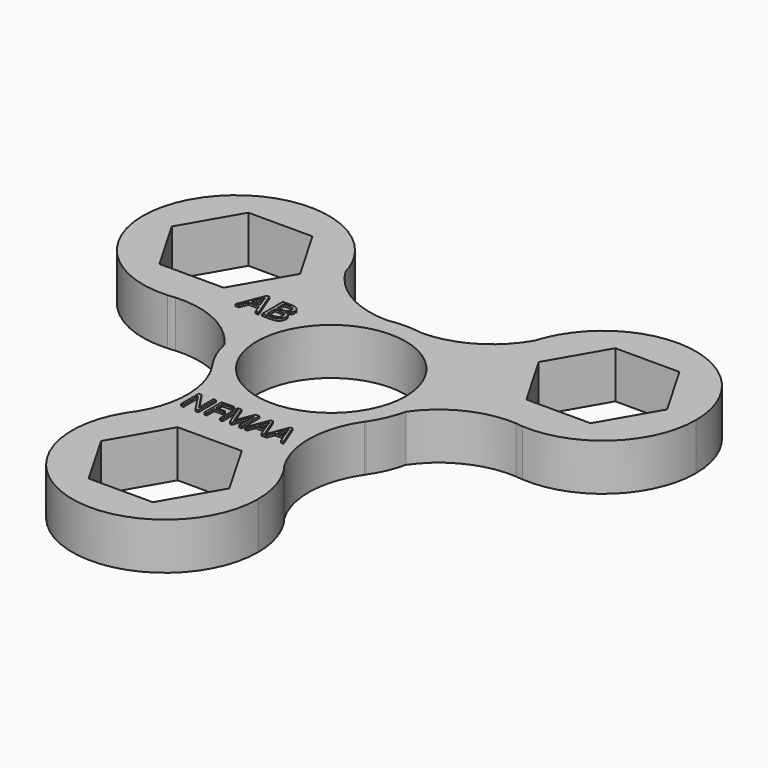
from build123d import *

# Parameters (mm, degrees)
F1_TEXT_SIZE = 4.5833333085
F2_DEPTH     = 7.3
F0_R         = 11.1353903362
F3_DEPTH     = 7
F4_TEXT_SIZE = 5.4166671665
F5_DEPTH     = 7.3


# Not quite as in the source:
# - Text() gives the source's letters only with a copy of the font that has no kerning and outlines rounded to 1/6400 em; it was checked with that copy


with BuildPart() as f2:
    # F1 (on Top) → F2 (new body)
    with BuildSketch(Plane.XY):
        with Locations((-8.2499992568, -18.2999996468)):
            Text('NFMAA', F1_TEXT_SIZE, font='Open Sans', text_align=(TextAlign.LEFT, TextAlign.BOTTOM))
    extrude(amount=F2_DEPTH)


with BuildPart() as f3:
    # F0 (on Top) → F3 (new body)
    with BuildSketch(Plane.XY):
        with BuildLine():
            ThreePointArc((13.5864677481, -3.0033933621), (13.8322264387, -1.5106254678), (13.9144700782, 0))
            ThreePointArc((13.9144700782, 0), (10.6851705077, 8.9128900351), (2.4961971103, 13.6887354253))
            ThreePointArc((2.4961971103, 13.6887354253), (1.2428155139, 13.7431823355), (0, 13.9144700782))
            ThreePointArc((0, 13.9144700782), (-1.2734696294, 13.7344813122), (-2.558322411, 13.6772608368))
            ThreePointArc((-2.558322411, 13.6772608368), (-11.6070934538, 7.6738425258), (-13.5864677481, -3.0033933621))
            ThreePointArc((-13.5864677481, -3.0033933621), (-12.2930583167, -5.3260981533), (-11.4830526526, -7.8582427638))
            ThreePointArc((-11.4830526526, -7.8582427638), (-11.4395938725, -7.9206308518), (-11.3964893616, -7.9832642313))
            ThreePointArc((-11.3964893616, -7.9832642313), (0, -13.9144700782), (11.3964893616, -7.9832642313))
            ThreePointArc((11.3964893616, -7.9832642313), (11.4395938725, -7.9206308518), (11.4830526526, -7.8582427638))
            ThreePointArc((11.4830526526, -7.8582427638), (12.2930583167, -5.3260981533), (13.5864677481, -3.0033933621))
        make_face()
        Circle(F0_R, mode=Mode.SUBTRACT)
        with BuildLine():
            ThreePointArc((2.4961971103, 13.6887354253), (10.6851705077, 8.9128900351), (13.9144700782, 0))
            ThreePointArc((13.9144700782, 0), (13.8322264387, -1.5106254678), (13.5864677481, -3.0033933621))
            ThreePointArc((13.5864677481, -3.0033933621), (18.7682974416, 1.4209787448), (25.4552118556, 2.7292612574))
            ThreePointArc((25.4552118556, 2.7292612574), (15.7241567662, 9.0088698377), (14.1162936282, 20.4780325449))
            ThreePointArc((14.1162936282, 20.4780325449), (9.2191414593, 15.5209334854), (2.4961971103, 13.6887354253))
        make_face()
        with BuildLine():
            ThreePointArc((0, 13.9144700782), (1.2428155139, 13.7431823355), (2.4961971103, 13.6887354253))
            ThreePointArc((2.4961971103, 13.6887354253), (1.2531915403, 13.8579215079), (0, 13.9144700782))
        make_face()
        with BuildLine():
            ThreePointArc((11.4830526526, -7.8582427638), (12.7676389343, -5.5317152493), (13.5864677481, -3.0033933621))
            ThreePointArc((13.5864677481, -3.0033933621), (12.2930583167, -5.3260981533), (11.4830526526, -7.8582427638))
        make_face()
        with BuildLine():
            ThreePointArc((-2.558322411, 13.6772608368), (-1.2734696294, 13.7344813122), (0, 13.9144700782))
            ThreePointArc((0, 13.9144700782), (-1.2846479851, 13.8550408556), (-2.558322411, 13.6772608368))
        make_face()
        with BuildLine():
            ThreePointArc((15.3229415527, 23.3225313582), (14.8017809107, 21.8654279382), (14.1162936282, 20.4780325449))
            ThreePointArc((14.1162936282, 20.4780325449), (15.7241567662, 9.0088698377), (25.4552118556, 2.7292612574))
            ThreePointArc((25.4552118556, 2.7292612574), (26.0018090129, 2.6832452791), (26.5460682638, 2.6149240491))
            ThreePointArc((26.5460682638, 2.6149240491), (36.9640624183, 6.3464255382), (41.3644709454, 16.5000017732))
            ThreePointArc((41.3644709454, 16.5000017732), (30.9763923364, 29.9602038803), (15.3229415527, 23.3225313582))
        make_face()
        Polygon((17.8500022739, 16.5000017732), (22.6500015706, 24.8138444314), (32.2500001639, 24.8138444314), (37.0499994606, 16.5000017732), (32.2500001639, 8.1861591151), (22.6500015706, 8.1861591151), align=None, mode=Mode.SUBTRACT)
        with BuildLine():
            ThreePointArc((15.3229415527, 23.3225313582), (14.6404164966, 21.9338793766), (14.1162936282, 20.4780325449))
            ThreePointArc((14.1162936282, 20.4780325449), (14.8017809107, 21.8654279382), (15.3229415527, 23.3225313582))
        make_face()
        with BuildLine():
            ThreePointArc((11.3964893616, -7.9832642313), (11.4399417956, -7.9208717494), (11.4830526526, -7.8582427638))
            ThreePointArc((11.4830526526, -7.8582427638), (11.4395938725, -7.9206308518), (11.3964893616, -7.9832642313))
        make_face()
        with BuildLine():
            ThreePointArc((26.5460682638, 2.6149240491), (26.0018090129, 2.6832452791), (25.4552118556, 2.7292612574))
            ThreePointArc((25.4552118556, 2.7292612574), (25.9995130184, 2.6613398958), (26.5460682638, 2.6149240491))
        make_face()
        with BuildLine():
            ThreePointArc((-13.5864677481, -3.0033933621), (-11.6070934538, 7.6738425258), (-2.558322411, 13.6772608368))
            ThreePointArc((-2.558322411, 13.6772608368), (-9.1702984419, 15.4459809359), (-14.0493052688, 20.2461778283))
            ThreePointArc((-14.0493052688, 20.2461778283), (-13.6645727729, 18.3906233146), (-13.5355307891, 16.5000017732))
            ThreePointArc((-13.5355307891, 16.5000017732), (-16.9293328853, 7.3935193145), (-25.4552118556, 2.7292612574))
            ThreePointArc((-25.4552118556, 2.7292612574), (-18.7682974416, 1.4209787448), (-13.5864677481, -3.0033933621))
        make_face()
        with BuildLine():
            ThreePointArc((11.0179525727, -22.5467241061), (9.0582471947, -15.2091375496), (11.3964893616, -7.9832642313))
            ThreePointArc((11.3964893616, -7.9832642313), (0, -13.9144700782), (-11.3964893616, -7.9832642313))
            ThreePointArc((-11.3964893616, -7.9832642313), (-9.0582471947, -15.2091375496), (-11.0179525727, -22.5467241061))
            ThreePointArc((-11.0179525727, -22.5467241061), (0, -17.1303243185), (11.0179525727, -22.5467241061))
        make_face()
        with BuildLine():
            ThreePointArc((-11.4830526526, -7.8582427638), (-12.2930583167, -5.3260981533), (-13.5864677481, -3.0033933621))
            ThreePointArc((-13.5864677481, -3.0033933621), (-12.7676389343, -5.5317152493), (-11.4830526526, -7.8582427638))
        make_face()
        with BuildLine():
            ThreePointArc((-15.4499762043, 23.5435722915), (-14.8602012518, 21.8479110397), (-14.0493052688, 20.2461778283))
            ThreePointArc((-14.0493052688, 20.2461778283), (-14.6430750062, 21.9401421709), (-15.4499762043, 23.5435722915))
        make_face()
        with BuildLine():
            ThreePointArc((-13.5355307891, 16.5000017732), (-13.6645727729, 18.3906233146), (-14.0493052688, 20.2461778283))
            ThreePointArc((-14.0493052688, 20.2461778283), (-14.8602012518, 21.8479110397), (-15.4499762043, 23.5435722915))
            ThreePointArc((-15.4499762043, 23.5435722915), (-39.7434994578, 23.0178518759), (-26.5460682638, 2.6149240491))
            ThreePointArc((-26.5460682638, 2.6149240491), (-26.0018090129, 2.6832452791), (-25.4552118556, 2.7292612574))
            ThreePointArc((-25.4552118556, 2.7292612574), (-16.9293328853, 7.3935193145), (-13.5355307891, 16.5000017732))
        make_face()
        Polygon((-22.6500015706, 24.8138444314), (-17.8500022739, 16.5000017732), (-22.6500015706, 8.1861591151), (-32.2500001639, 8.1861591151), (-37.0499994606, 16.5000017732), (-32.2500001639, 24.8138444314), align=None, mode=Mode.SUBTRACT)
        with BuildLine():
            ThreePointArc((-11.4830526526, -7.8582427638), (-11.4399417956, -7.9208717494), (-11.3964893616, -7.9832642313))
            ThreePointArc((-11.3964893616, -7.9832642313), (-11.4395938725, -7.9206308518), (-11.4830526526, -7.8582427638))
        make_face()
        with BuildLine():
            ThreePointArc((11.8627967872, -23.7724818387), (11.4233595269, -23.1713305375), (11.0179525727, -22.5467241061))
            ThreePointArc((11.0179525727, -22.5467241061), (0, -17.1303243185), (-11.0179525727, -22.5467241061))
            ThreePointArc((-11.0179525727, -22.5467241061), (-11.4233595269, -23.1713305375), (-11.8627967872, -23.7724818387))
            ThreePointArc((-11.8627967872, -23.7724818387), (-3.7780912255, -44.4365270795), (13.9144700782, -31.0447943966))
            ThreePointArc((13.9144700782, -31.0447943966), (13.3917326828, -27.2667031711), (11.8627967872, -23.7724818387))
        make_face()
        Polygon((4.7999992967, -22.7309517385), (9.5999985933, -31.0447943966), (4.7999992967, -39.3586370548), (-4.7999992967, -39.3586370548), (-9.5999985933, -31.0447943966), (-4.7999992967, -22.7309517385), align=None, mode=Mode.SUBTRACT)
        with BuildLine():
            ThreePointArc((11.8627967872, -23.7724818387), (11.4567793608, -23.1482961706), (11.0179525727, -22.5467241061))
            ThreePointArc((11.0179525727, -22.5467241061), (11.4233595269, -23.1713305375), (11.8627967872, -23.7724818387))
        make_face()
        with BuildLine():
            ThreePointArc((-26.5460682638, 2.6149240491), (-25.9995130184, 2.6613398958), (-25.4552118556, 2.7292612574))
            ThreePointArc((-25.4552118556, 2.7292612574), (-26.0018090129, 2.6832452791), (-26.5460682638, 2.6149240491))
        make_face()
        with BuildLine():
            ThreePointArc((-11.8627967872, -23.7724818387), (-11.4233595269, -23.1713305375), (-11.0179525727, -22.5467241061))
            ThreePointArc((-11.0179525727, -22.5467241061), (-11.4567793608, -23.1482961706), (-11.8627967872, -23.7724818387))
        make_face()
    extrude(amount=F3_DEPTH)

    # F4 (on Top) → F5 (join)
    with BuildSketch(Plane.XY):
        with Locations((-18.6000056565, 5.3999982774)):
            Text('AB', F4_TEXT_SIZE, font='Open Sans', text_align=(TextAlign.LEFT, TextAlign.BOTTOM))
    extrude(amount=F5_DEPTH)


solid = Compound([f2.part, f3.part])
